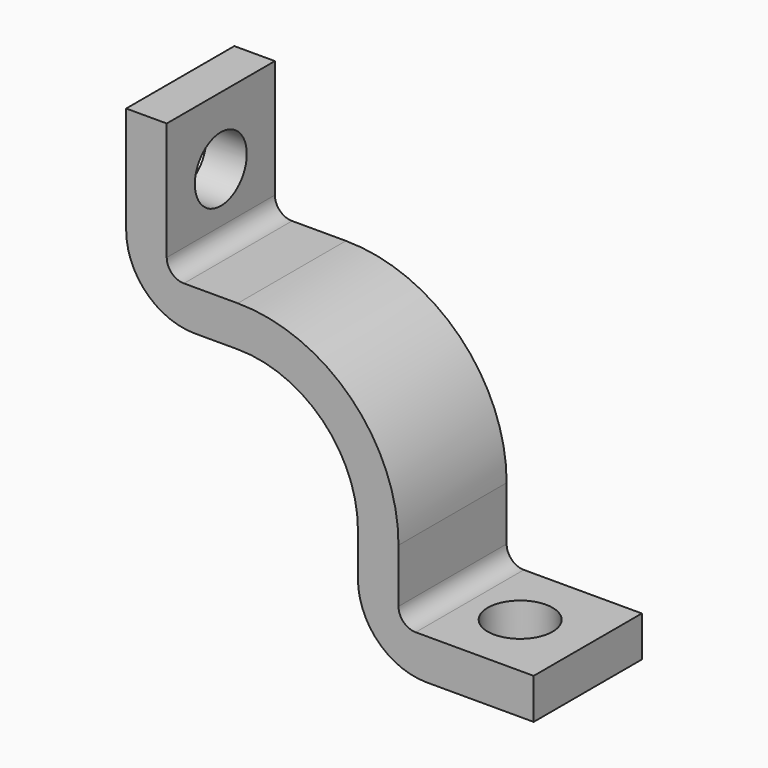
from build123d import *

# Parameters (mm, degrees)
F1_DEPTH = 10
F2_R     = 2.4
F3_DEPTH = 3
F7_R     = 5.08
F8_R     = 1.27


# Not quite as in the source:
# - a pattern or mirror of a feature is missing from the dataset's text; its kind, count and spacing are read off the source's solid


with BuildPart() as f1:
    # F0 (on Front) → F1 (new body)
    with BuildSketch(Plane.XZ):
        with BuildLine():
            ThreePointArc((0, 8.89), (6.2861792847, 6.2861792847), (8.89, 0))
            Line((8.89, 0), (8.89, -8.255))
            Line((8.89, -8.255), (21.89, -8.255))
            Line((21.89, -8.255), (21.89, -5.255))
            Line((21.89, -5.255), (11.89, -5.255))
            Line((11.89, -5.255), (11.89, 0))
            ThreePointArc((11.89, 0), (8.4074996283, 8.4074996283), (0, 11.89))
            Line((0, 11.89), (-5.255, 11.89))
            Line((-5.255, 11.89), (-5.255, 21.89))
            Line((-5.255, 21.89), (-8.255, 21.89))
            Line((-8.255, 21.89), (-8.255, 8.89))
            Line((-8.255, 8.89), (0, 8.89))
        make_face()
    extrude(amount=F1_DEPTH)

    # F2 (on face) → F3 (cut, through all)
    with BuildSketch(Plane.XY.offset(-5.255)):
        with Locations((16.89, -5)):
            Circle(F2_R)
    f3 = extrude(amount=-F3_DEPTH, mode=Mode.SUBTRACT)

    # F3_copies: F3 across plane
    add(f3.mirror(Plane(origin=(0, 0, 0), x_dir=(-0.7071067812, 0, -0.7071067812), z_dir=(-0.7071067812, 0, 0.7071067812))), mode=Mode.SUBTRACT)

    # F7
    f7_edges = [f1.edges().sort_by_distance(p)[0] for p in [
        (-8.255, -5, 8.89),
        (8.89, -5, -8.255),
    ]]
    fillet(f7_edges, radius=F7_R)

    # F8
    f8_edges = [f1.edges().sort_by_distance(p)[0] for p in [
        (-5.255, -5, 11.89),
        (11.89, -5, -5.255),
    ]]
    fillet(f8_edges, radius=F8_R)


solid = f1.part
